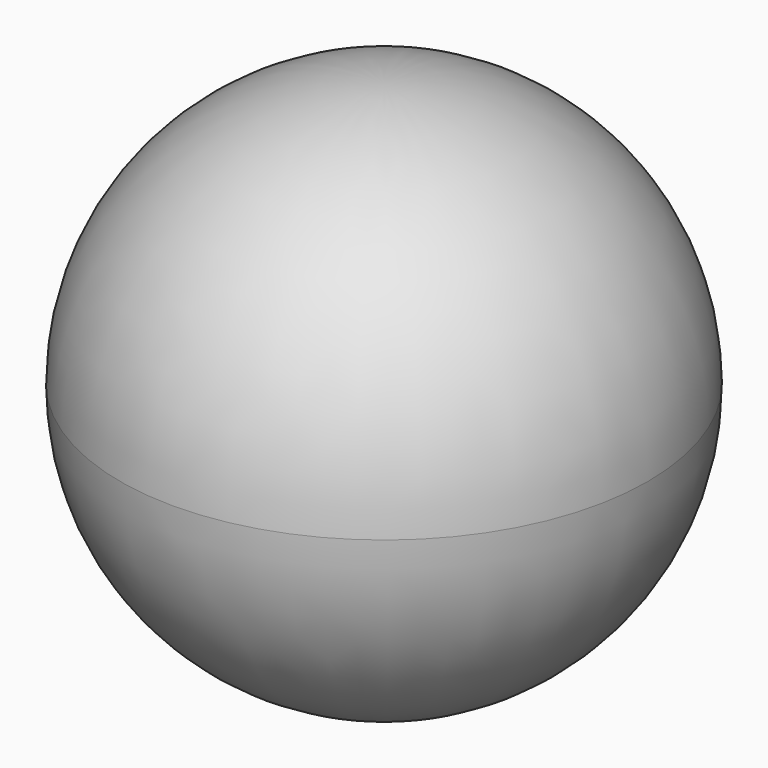
from build123d import *

# Parameters (mm, degrees)
F0_R     = 76.2
F1_DEPTH = 76.2
F2_R     = 76.19999


# Not quite as in the source:
# - a fillet or chamfer is up to 0.001 mm smaller than in the source, because OpenCascade refuses the exact size


with BuildPart() as f1:
    # F0 (on Top) → F1 (new body, symmetric)
    with BuildSketch(Plane.XY):
        Circle(F0_R)
    extrude(amount=F1_DEPTH, both=True)

    # F2 (radius 76.2 in the source; OpenCascade refuses exactly that, so slightly less here)
    f2_edges = [f1.edges().sort_by_distance(p)[0] for p in [
        (-76.2, 0, 76.2),
        (-76.2, 0, -76.2),
    ]]
    fillet(f2_edges, radius=F2_R)


solid = f1.part
